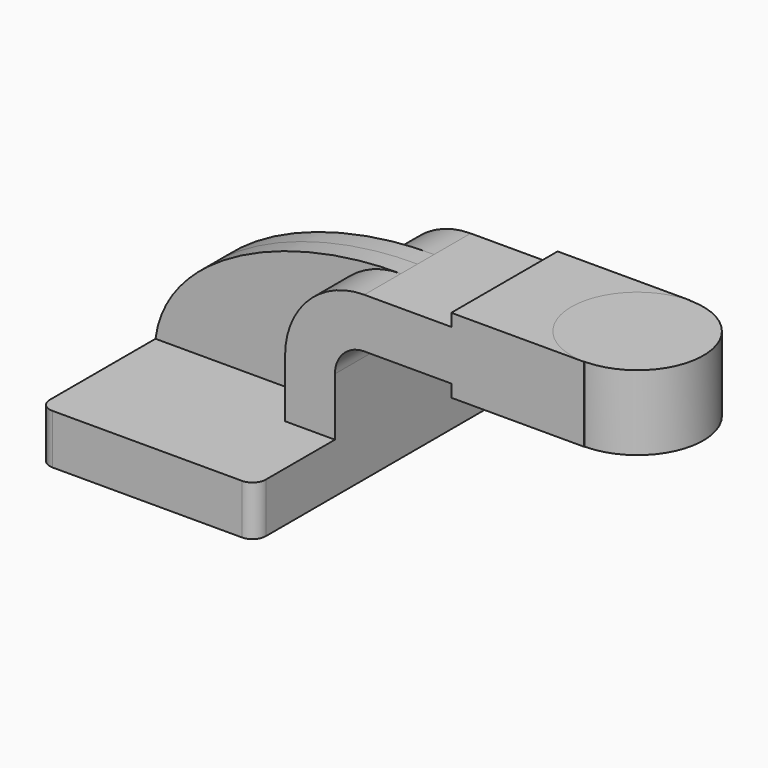
from build123d import *

# Parameters (mm, degrees)
F1_DEPTH = 63.5
F0_W     = 25.5705659628
F0_H     = 4.7498
F0_H_2   = 19.05
F0_H_3   = 4.7752
F2_DEPTH = 25.4
F3_DEPTH = 7.9375
F5_R     = 5.08


with BuildPart() as f1:
    # F0 (on Front) → F1 (new body, symmetric)
    with BuildSketch(Plane.XZ):
        Polygon((22.225, 9.525), (-41.275, 9.525), (-41.275, -9.525), (41.275, -9.525), (41.275, 9.525), align=None)
    extrude(amount=F1_DEPTH, both=True)

    # F0 (on Front) → F2 (join, symmetric)
    with BuildSketch(Plane.XZ):
        Polygon((111.2955659628, 66.675), (111.2955659628, 61.9252), (111.2955659628, 42.8752), (111.2955659628, 38.1), (136.525, 38.1), (136.525, 66.675), align=None)
        with Locations((98.5102829814, 64.3001)):
            Rectangle(F0_W, F0_H)
        with Locations((98.5102829814, 52.4002)):
            Rectangle(F0_W, F0_H_2)
        with Locations((98.5102829814, 40.4876)):
            Rectangle(F0_W, F0_H_3)
        with BuildLine():
            Line((22.225, 31.6498798487), (22.225, 9.525))
            Line((22.225, 9.525), (41.275, 9.525))
            Line((41.275, 9.525), (41.275, 31.6498798487))
            ThreePointArc((41.275, 31.6498798487), (44.5628201513, 39.5873798487), (52.5003201513, 42.8752))
            Line((52.5003201513, 42.8752), (85.725, 42.8752))
            Line((85.725, 42.8752), (85.725, 61.9252))
            Line((85.725, 61.9252), (52.5003201513, 61.9252))
            ThreePointArc((52.5003201513, 61.9252), (31.0924359697, 53.0577640303), (22.225, 31.6498798487))
        make_face()
    extrude(amount=F2_DEPTH, both=True)

    # F0 (on Front) → F3 (join, symmetric)
    with BuildSketch(Plane.XZ):
        with BuildLine():
            add(Edge.make_bspline(
                [(-41.275, 9.525), (-37.0544083416, 41.9974066317), (9.7774779424, 62.3142682016), (52.5003201513, 61.9252)],
                knots=[0, 0, 0, 0, 107.4224912648, 107.4224912648, 107.4224912648, 107.4224912648], degree=3))
            Line((-41.275, 9.525), (22.225, 9.525))
            Line((22.225, 9.525), (22.225, 31.6498798487))
            ThreePointArc((22.225, 31.6498798487), (31.0924359697, 53.0577640303), (52.5003201513, 61.9252))
        make_face()
    extrude(amount=F3_DEPTH, both=True)

    # F5
    f5_edges = [f1.edges().sort_by_distance(p)[0] for p in [
        (41.275, -63.5, 0),
        (-41.275, -63.5, 0),
        (-41.275, 63.5, 0),
        (41.275, 63.5, 0),
    ]]
    fillet(f5_edges, radius=F5_R)


with BuildPart() as f4:
    # F0 (on Front) → F4 (revolve)
    with BuildSketch(Plane.XZ):
        Polygon((111.2955659628, 66.675), (111.2955659628, 61.9252), (111.2955659628, 42.8752), (111.2955659628, 38.1), (136.525, 38.1), (136.525, 66.675), align=None)
    revolve(axis=Axis((136.525, 0, 52.3875), (0, 0, 1)))


solid = Compound([f1.part, f4.part])
